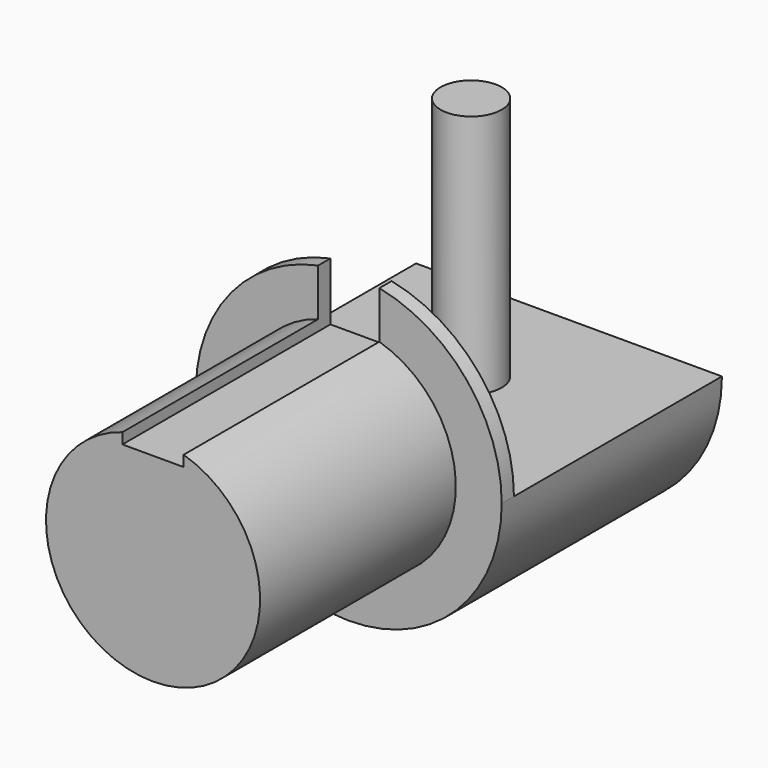
from build123d import *

# Parameters (mm, degrees)
F0_R     = 5
F1_DEPTH = 9
F2_R     = 3.5
F3_DEPTH = 8
F4_W     = 9.3990088471
F4_H     = 6
F5_DEPTH = 12.5
F7_DEPTH = 25
F8_R     = 1
F9_DEPTH = 8


with BuildPart() as f1:
    # F0 (on Front) → F1 (new body)
    with BuildSketch(Plane.XZ):
        Circle(F0_R)
    extrude(amount=F1_DEPTH)

    # F2 (on face) → F3 (join)
    with BuildSketch(Plane.XZ.offset(9)):
        Circle(F2_R)
    extrude(amount=F3_DEPTH)

    # F4 (on Right) → F5 (cut, symmetric)
    with BuildSketch(Plane.YZ):
        with Locations((-3.8004955764, 3)):
            Rectangle(F4_W, F4_H)
    extrude(amount=F5_DEPTH, both=True, mode=Mode.SUBTRACT)

    # F6 (on face) → F7 (cut)
    with BuildSketch(Plane(origin=(0, -8.5, 0), x_dir=(-1, 0, 0), z_dir=(0, 1, 0))):
        with BuildLine():
            Line((-1, 3), (1, 3))
            Line((1, 3), (1, 4.8989794856))
            ThreePointArc((1, 4.8989794856), (0, 5), (-1, 4.8989794856))
            Line((-1, 4.8989794856), (-1, 3))
        make_face()
    extrude(amount=-F7_DEPTH, mode=Mode.SUBTRACT)

    # F8 (on face) → F9 (join)
    with BuildSketch(Plane.XY):
        with Locations((0, -4)):
            Circle(F8_R)
    extrude(amount=F9_DEPTH)


solid = f1.part
